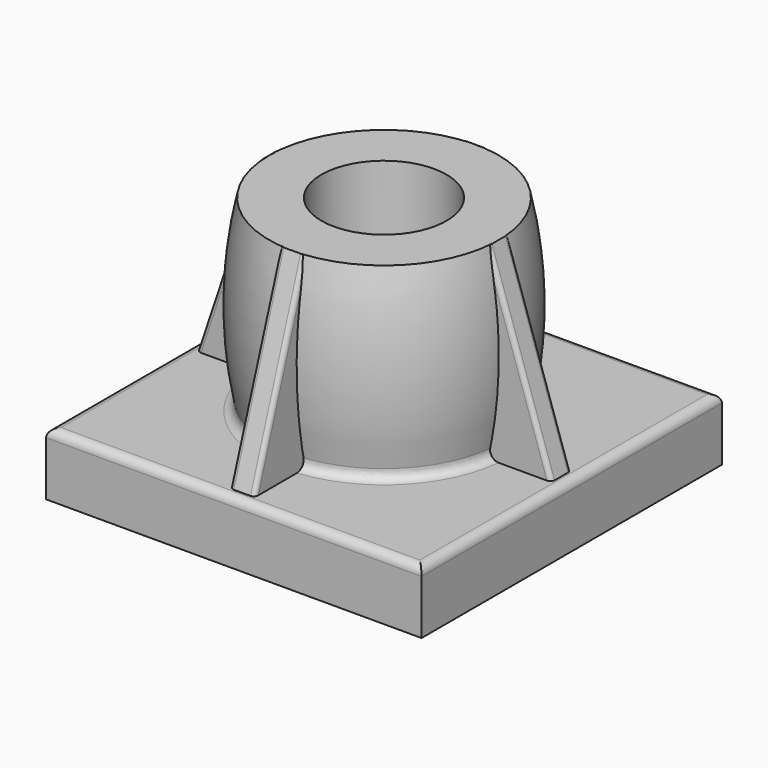
from build123d import *

# Parameters (mm, degrees)
F0_W           = 90
F0_H           = 90
F1_DEPTH       = 15
F5_DEPTH       = 3
F7_COUNT       = 4
F8_R           = 2
F9_T1_DEPTH    = 52.4341649025
F10_T1_DEPTH   = 52.4341649025
F10_2_T1_DEPTH = 52.4341649025
F10_3_T1_DEPTH = 52.4341649025


# Not quite as in the source:
# - a fillet or chamfer that OpenCascade refuses, or shapes differently, is made with other operations: its cross-section is extruded or revolved along the edge and cut away or added


with BuildPart() as f1:
    # F0 (on Top) → F1 (new body)
    with BuildSketch(Plane.XY):
        Rectangle(F0_W, F0_H)
    extrude(amount=F1_DEPTH)

    # F2 (on Front) → F3 (revolve)
    with BuildSketch(Plane.XZ):
        with BuildLine():
            Line((-27.5, 15), (-15, 15))
            Line((-15, 15), (-15, 60))
            Line((-15, 60), (-27.5, 60))
            ThreePointArc((-27.5, 60), (-30.0641236505, 37.5), (-27.5, 15))
        make_face()
    revolve(axis=Axis((0, 0, 27.5), (0, 0, 1)))


with BuildPart() as f5:
    # F4 (on Front) → F5 (new body, symmetric)
    with BuildSketch(Plane.XZ):
        Polygon((-42.5, 15), (-22.5, 15), (-22.5, 60), (-27.5, 60), align=None)
    extrude(amount=F5_DEPTH, both=True)

    # F6: cut F1
    add(f1.part, mode=Mode.SUBTRACT)


with BuildPart() as f7_1:
    # F7: instance of F5
    add(f5.part.rotate(Axis((0, 0, 27.5), (0, 0, 1)), 1 * 360 / F7_COUNT))

    # F10#3: fillet of radius 1 on 2 edges, made by hand

    # F10_3_s2 → F10_3_t1 (cut)
    with BuildSketch(Plane(origin=(0, 16.040569415, 48.1217082451), x_dir=(1, 0, 0), z_dir=(0, -0.316227766, -0.9486832981))):
        with BuildLine():
            ThreePointArc((3, 44.0624566574), (2.7071067812, 44.7695634386), (2, 45.0624566574))
            Line((2, 45.0624566574), (3, 45.0624566574))
            Line((3, 45.0624566574), (3, 44.0624566574))
        make_face()
        with BuildLine():
            ThreePointArc((-3, 44.0624566574), (-2.7071067812, 44.7695634386), (-2, 45.0624566574))
            Line((-2, 45.0624566574), (-3, 45.0624566574))
            Line((-3, 45.0624566574), (-3, 44.0624566574))
        make_face()
    extrude(amount=F10_3_T1_DEPTH, mode=Mode.SUBTRACT)


with BuildPart() as f7_2:
    # F7: instance of F5
    add(f5.part.rotate(Axis((0, 0, 27.5), (0, 0, 1)), 2 * 360 / F7_COUNT))

    # F10#2: fillet of radius 1 on 2 edges, made by hand

    # F10_2_s2 → F10_2_t1 (cut)
    with BuildSketch(Plane(origin=(-16.040569415, 0, 48.1217082451), x_dir=(0, 1, 0), z_dir=(0.316227766, 0, -0.9486832981))):
        with BuildLine():
            ThreePointArc((-3, 44.0624566574), (-2.7071067812, 44.7695634386), (-2, 45.0624566574))
            Line((-2, 45.0624566574), (-3, 45.0624566574))
            Line((-3, 45.0624566574), (-3, 44.0624566574))
        make_face()
        with BuildLine():
            ThreePointArc((3, 44.0624566574), (2.7071067812, 44.7695634386), (2, 45.0624566574))
            Line((2, 45.0624566574), (3, 45.0624566574))
            Line((3, 45.0624566574), (3, 44.0624566574))
        make_face()
    extrude(amount=F10_2_T1_DEPTH, mode=Mode.SUBTRACT)


with BuildPart() as f7_3:
    # F7: instance of F5
    add(f5.part.rotate(Axis((0, 0, 27.5), (0, 0, 1)), 3 * 360 / F7_COUNT))

    # F10: fillet of radius 1 on 2 edges, made by hand

    # F10_s2 → F10_t1 (cut)
    with BuildSketch(Plane(origin=(0, -16.040569415, 48.1217082451), x_dir=(1, 0, 0), z_dir=(0, 0.316227766, -0.9486832981))):
        with BuildLine():
            ThreePointArc((-3, -44.0624566574), (-2.7071067812, -44.7695634386), (-2, -45.0624566574))
            Line((-2, -45.0624566574), (-3, -45.0624566574))
            Line((-3, -45.0624566574), (-3, -44.0624566574))
        make_face()
        with BuildLine():
            ThreePointArc((3, -44.0624566574), (2.7071067812, -44.7695634386), (2, -45.0624566574))
            Line((2, -45.0624566574), (3, -45.0624566574))
            Line((3, -45.0624566574), (3, -44.0624566574))
        make_face()
    extrude(amount=F10_T1_DEPTH, mode=Mode.SUBTRACT)


with BuildPart() as f1_1:
    add(f1.part)

    # F8
    f8_edges = [f1_1.edges().sort_by_distance(p)[0] for p in [
        (45, 0, 15),
        (0, -45, 15),
        (0, 45, 15),
        (-45, 0, 15),
        (27.5, 0, 15),
    ]]
    fillet(f8_edges, radius=F8_R)


with BuildPart() as f5_1:
    add(f5.part)

    # F9: fillet of radius 1 on 2 edges, made by hand

    # F9_s2 → F9_t1 (cut)
    with BuildSketch(Plane(origin=(16.040569415, 0, 48.1217082451), x_dir=(0, 1, 0), z_dir=(-0.316227766, 0, -0.9486832981))):
        with BuildLine():
            ThreePointArc((3, -44.0624566574), (2.7071067812, -44.7695634386), (2, -45.0624566574))
            Line((2, -45.0624566574), (3, -45.0624566574))
            Line((3, -45.0624566574), (3, -44.0624566574))
        make_face()
        with BuildLine():
            ThreePointArc((-3, -44.0624566574), (-2.7071067812, -44.7695634386), (-2, -45.0624566574))
            Line((-2, -45.0624566574), (-3, -45.0624566574))
            Line((-3, -45.0624566574), (-3, -44.0624566574))
        make_face()
    extrude(amount=F9_T1_DEPTH, mode=Mode.SUBTRACT)


solid = Compound([f7_1.part, f7_2.part, f7_3.part, f1_1.part, f5_1.part])
